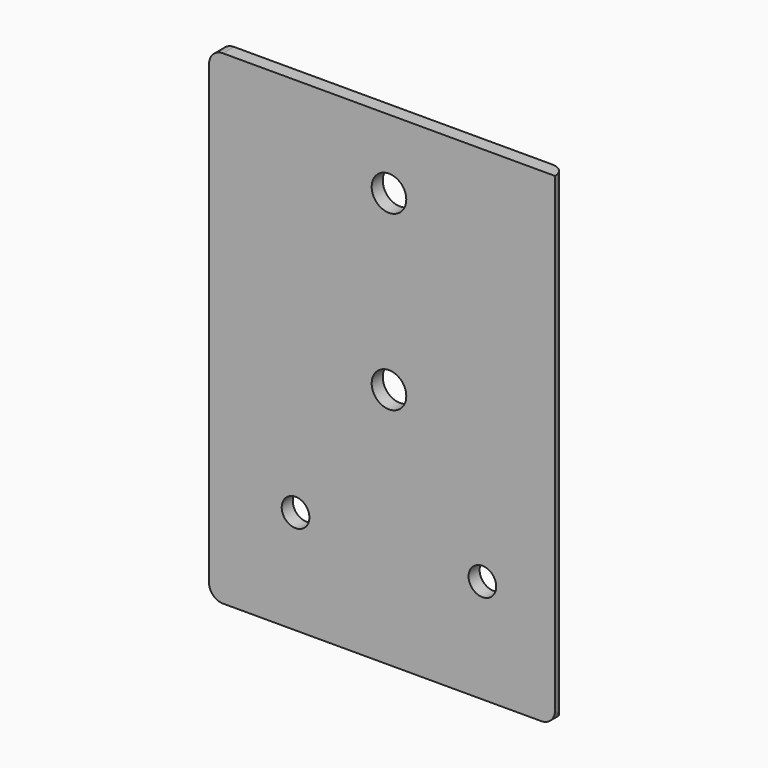
from build123d import *

# Parameters (mm, degrees)
F0_W     = 50
F0_H     = 70
F1_DEPTH = 2
F2_R     = 1.99999
F3_R     = 2
F3_R_2   = 2.5
F4_DEPTH = 2.001


# Not quite as in the source:
# - a fillet or chamfer is up to 0.001 mm smaller than in the source, because OpenCascade refuses the exact size


with BuildPart() as f1:
    # F0 (on Front) → F1 (new body)
    with BuildSketch(Plane.XZ):
        with Locations((25, 35)):
            Rectangle(F0_W, F0_H)
    extrude(amount=F1_DEPTH)

    # F2 (radius 2 in the source; OpenCascade refuses exactly that, so slightly less here)
    f2_edges = [f1.edges().sort_by_distance(p)[0] for p in [
        (0, -1, 0),
        (50, -1, 0),
        (50, 0, 35),
        (0, -1, 70),
    ]]
    fillet(f2_edges, radius=F2_R)

    # F3 (on face) → F4 (cut, through all)
    with BuildSketch(Plane.XZ.offset(2)):
        with Locations((12.5, 15)):
            Circle(F3_R)
        with Locations((39.5, 15)):
            Circle(F3_R)
        with Locations((26, 60)):
            Circle(F3_R_2)
        with Locations((26, 35)):
            Circle(F3_R_2)
    extrude(amount=-F4_DEPTH, mode=Mode.SUBTRACT)


solid = f1.part
